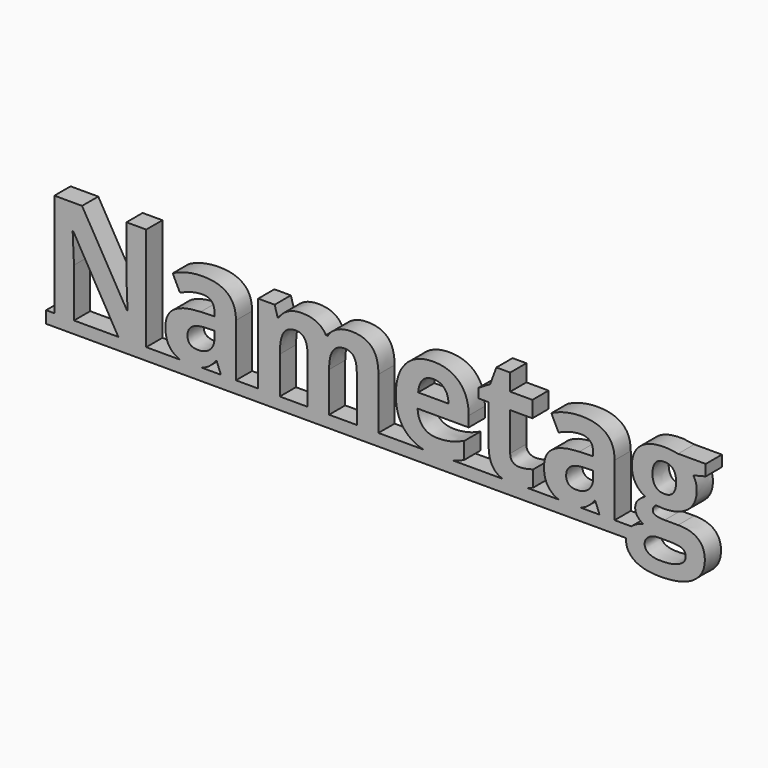
from build123d import *

# Parameters (mm, degrees)
F0_TEXT_SIZE = 21.5241810722
F1_DEPTH     = 3
F2_W         = 87.7251885831
F2_H         = 1.7831965815
F3_DEPTH     = 3


# Not quite as in the source:
# - Text() gives the source's letters only with a copy of the font that has no kerning and outlines rounded to 1/6400 em; it was checked with that copy


with BuildPart() as f1:
    # F0 (on Front) → F1 (new body)
    with BuildSketch(Plane.XZ):
        with Locations((-50, 0)):
            Text('Nametag', F0_TEXT_SIZE, font='Open Sans', font_style=FontStyle.BOLD, text_align=(TextAlign.LEFT, TextAlign.BOTTOM))
    extrude(amount=F1_DEPTH)

    # F2 (on face) → F3 (join)
    with BuildSketch(Plane.XZ.offset(3)):
        with Locations((-5.435148254, -0.8915982908)):
            Rectangle(F2_W, F2_H)
    extrude(amount=-F3_DEPTH)


solid = f1.part
